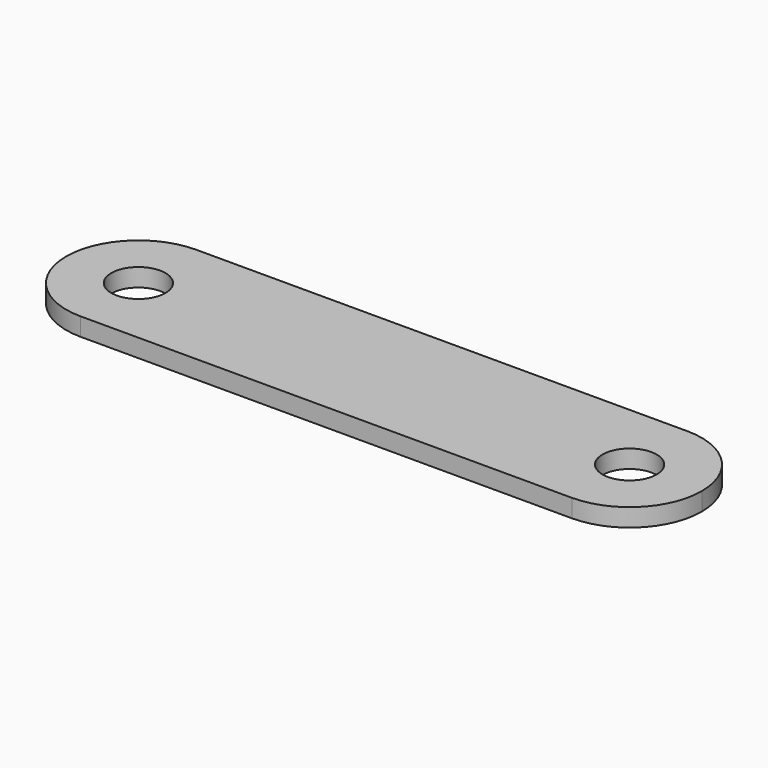
from build123d import *

# Parameters (mm, degrees)
F1_DEPTH = 3.175


# Not quite as in the source:
# - a length typed as a fraction of an inch, garbled in the dataset ("3 / 203.2 mm" for 3/8 in), is restored


with BuildPart() as f1:
    # F0 (on Top) → F1 (new body)
    with BuildSketch(Plane.XY):
        with BuildLine():
            ThreePointArc((-41.4974734498, 12.7), (-32.5172173287, 8.9802561211), (-28.7974734498, 0))
            Line((-28.7974734498, 0), (32.2387265502, 0))
            ThreePointArc((32.2387265502, 0), (35.9584704291, 8.9802561211), (44.9387265502, 12.7))
            Line((44.9387265502, 12.7), (-41.4974734498, 12.7))
        make_face()
        with BuildLine():
            ThreePointArc((-41.4974734498, -4.7625), (-44.8650694952, 3.3675960454), (-36.7349734498, 0))
            Line((-36.7349734498, 0), (-28.7974734498, 0))
            ThreePointArc((-28.7974734498, 0), (-32.5172173287, 8.9802561211), (-41.4974734498, 12.7))
            ThreePointArc((-41.4974734498, 12.7), (-54.1974734498, 0), (-41.4974734498, -12.7))
            Line((-41.4974734498, -12.7), (-41.4974734498, -4.7625))
        make_face()
        with BuildLine():
            Line((-28.7974734498, 0), (-36.7349734498, 0))
            ThreePointArc((-36.7349734498, 0), (-38.1298774044, -3.3675960454), (-41.4974734498, -4.7625))
            Line((-41.4974734498, -4.7625), (-41.4974734498, -12.7))
            ThreePointArc((-41.4974734498, -12.7), (-32.5172173287, -8.9802561211), (-28.7974734498, 0))
        make_face()
        with BuildLine():
            Line((32.2387265502, 0), (-28.7974734498, 0))
            ThreePointArc((-28.7974734498, 0), (-32.5172173287, -8.9802561211), (-41.4974734498, -12.7))
            Line((-41.4974734498, -12.7), (44.9387265502, -12.7))
            ThreePointArc((44.9387265502, -12.7), (35.9584704291, -8.9802561211), (32.2387265502, 0))
        make_face()
        with BuildLine():
            ThreePointArc((44.9387265502, 12.7), (35.9584704291, 8.9802561211), (32.2387265502, 0))
            ThreePointArc((32.2387265502, 0), (35.9584704291, -8.9802561211), (44.9387265502, -12.7))
            ThreePointArc((44.9387265502, -12.7), (53.9189826713, -8.9802561211), (57.6387265502, 0))
            ThreePointArc((57.6387265502, 0), (53.9189826713, 8.9802561211), (44.9387265502, 12.7))
        make_face()
        with BuildLine():
            ThreePointArc((49.7012265502, 0), (44.9387265502, -4.7625), (40.1762265502, 0))
            ThreePointArc((40.1762265502, 0), (44.9387265502, 4.7625), (49.7012265502, 0))
        make_face(mode=Mode.SUBTRACT)
    extrude(amount=F1_DEPTH)


solid = f1.part
